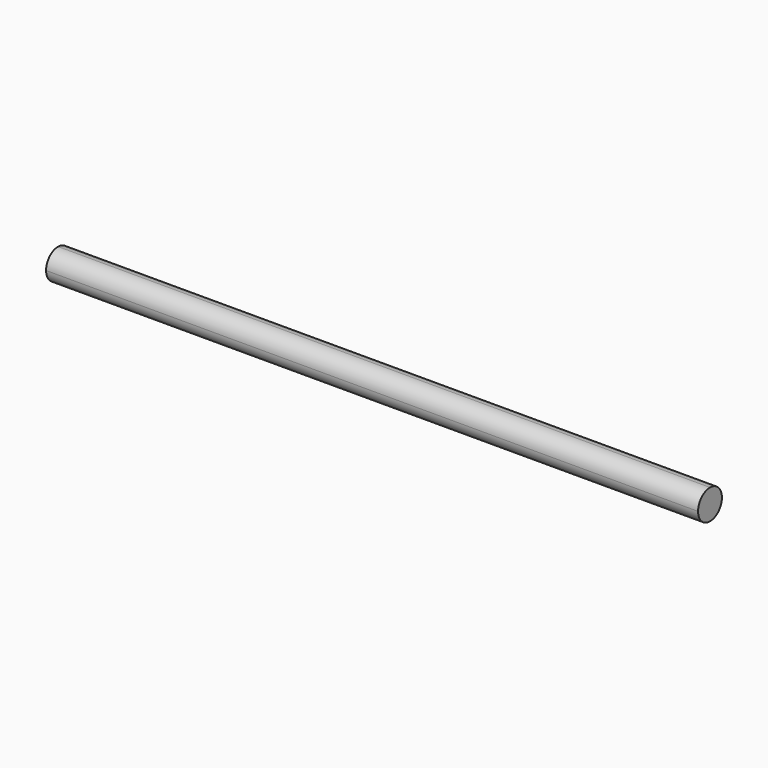
from build123d import *

# Parameters (mm, degrees)
F0_W     = 350
F0_H     = 16
F1_DEPTH = 16
F2_R     = 7.99999


# Not quite as in the source:
# - a fillet or chamfer is up to 0.001 mm smaller than in the source, because OpenCascade refuses the exact size
# - a feature names something its author has since deleted; it is built from what else it names


with BuildPart() as f1:
    # F0 (on Front) → F1 (new body)
    with BuildSketch(Plane.XZ):
        with Locations((175, -8)):
            Rectangle(F0_W, F0_H)
    extrude(amount=F1_DEPTH)

    # F2 (radius 8 in the source; OpenCascade refuses exactly that, so slightly less here)
    f2_edges = [f1.edges().sort_by_distance(p)[0] for p in [
        (175, -16, 0),
        (175, -16, -16),
        (175, 0, -16),
        (175, 0, 0),
    ]]
    fillet(f2_edges, radius=F2_R)


solid = f1.part
